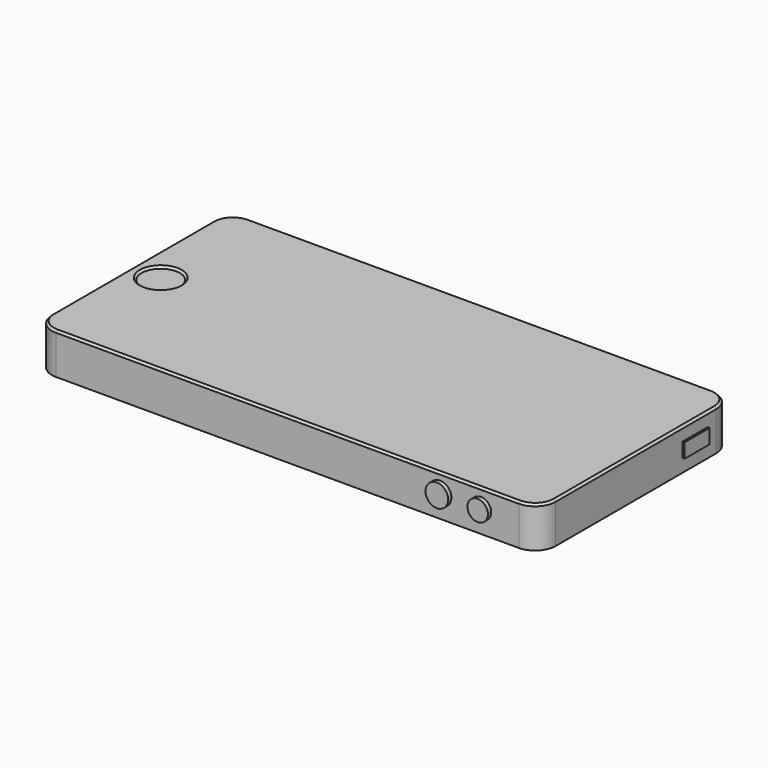
from build123d import *

# Parameters (mm, degrees)
F0_W     = 123
F0_H     = 59
F1_DEPTH = 10
F2_R     = 5
F3_R     = 5
F4_R     = 2.7669489105
F4_R_2   = 2.5059208377
F5_DEPTH = 1
F6_W     = 7.6256990433
F6_H     = 3.5195555538
F7_DEPTH = 0.5
F8_R     = 4.6382964955
F9_DEPTH = 0.5
F10_SIZE = 0.49999


# Not quite as in the source:
# - a fillet or chamfer is up to 0.001 mm smaller than in the source, because OpenCascade refuses the exact size


with BuildPart() as f1:
    # F0 (on Top) → F1 (new body)
    with BuildSketch(Plane.XY):
        Rectangle(F0_W, F0_H)
    extrude(amount=F1_DEPTH)

    # F2
    f2_edges = [f1.edges().sort_by_distance(p)[0] for p in [
        (-61.5, 29.5, 5),
        (61.5, 29.5, 5),
    ]]
    fillet(f2_edges, radius=F2_R)

    # F3
    f3_edges = [f1.edges().sort_by_distance(p)[0] for p in [
        (-61.5, -29.5, 5),
        (61.5, -29.5, 5),
    ]]
    fillet(f3_edges, radius=F3_R)

    # F4 (on face) → F5 (join)
    with BuildSketch(Plane.XZ.offset(29.5)):
        with Locations((37.291161716, 5.468532443)):
            Circle(F4_R)
        with Locations((47.2632274032, 5.468532443)):
            Circle(F4_R_2)
    extrude(amount=F5_DEPTH)

    # F6 (on face) → F7 (join)
    with BuildSketch(Plane.YZ.offset(61.5)):
        with Locations((18.0802661926, 4.9434783868)):
            Rectangle(F6_W, F6_H)
    extrude(amount=F7_DEPTH)

    # F8 (on face) → F9 (cut)
    with BuildSketch(Plane.XY.offset(10)):
        with Locations((-54.5105189085, 0)):
            Circle(F8_R)
    extrude(amount=-F9_DEPTH, mode=Mode.SUBTRACT)

    # F10 (size 0.5 in the source; OpenCascade refuses exactly that, so slightly less here)
    f10_edges = [f1.edges().sort_by_distance(p)[0] for p in [
        (61.5, 0, 10),
        (60.035534, -28.035534, 10),
        (60.035534, 28.035534, 10),
        (0, -29.5, 10),
        (0, 29.5, 10),
        (-60.035534, -28.035534, 10),
        (-60.035534, 28.035534, 10),
        (-61.5, 0, 10),
        (-59.148815, 0, 10),
    ]]
    chamfer(f10_edges, length=F10_SIZE)


solid = f1.part
